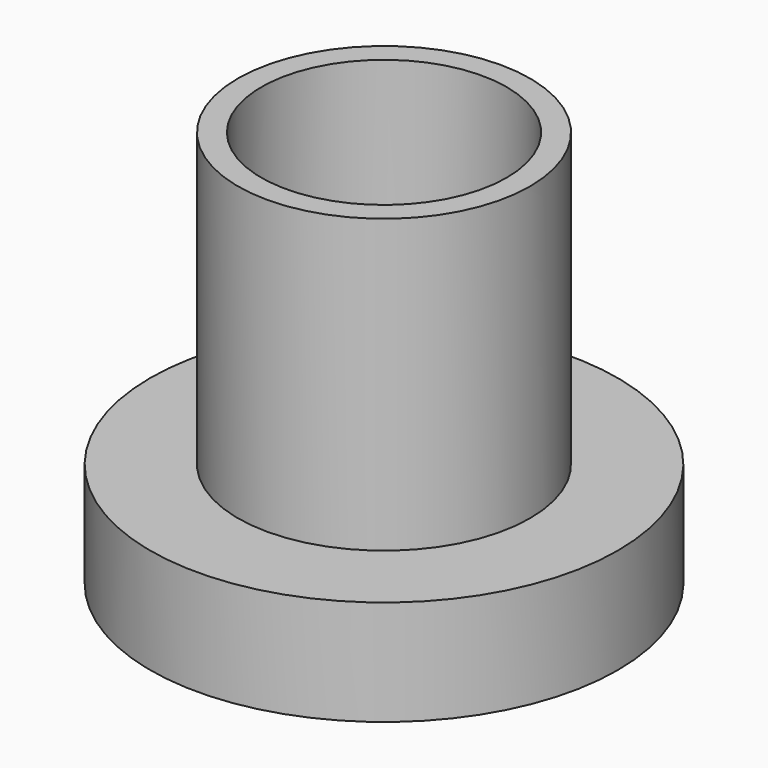
from build123d import *

# Parameters (mm, degrees)
F0_R     = 5
F1_DEPTH = 3.2
F2_R     = 5
F2_R_2   = 4.2
F3_DEPTH = 6.8
F4_R     = 8
F4_R_2   = 5
F5_DEPTH = 3.6


with BuildPart() as f1:
    # F0 (on Top) → F1 (new body)
    with BuildSketch(Plane.XY):
        Circle(F0_R)
    extrude(amount=F1_DEPTH)

    # F2 (on face) → F3 (join)
    with BuildSketch(Plane.XY.offset(3.2)):
        Circle(F2_R)
        Circle(F2_R_2, mode=Mode.SUBTRACT)
    extrude(amount=F3_DEPTH)

    # F4 (on face) → F5 (join)
    with BuildSketch(Plane(origin=(0, 0, 0), x_dir=(1, 0, 0), z_dir=(0, 0, -1))):
        Circle(F4_R)
        Circle(F4_R_2, mode=Mode.SUBTRACT)
        Circle(F4_R_2)
    extrude(amount=F5_DEPTH)


solid = f1.part
